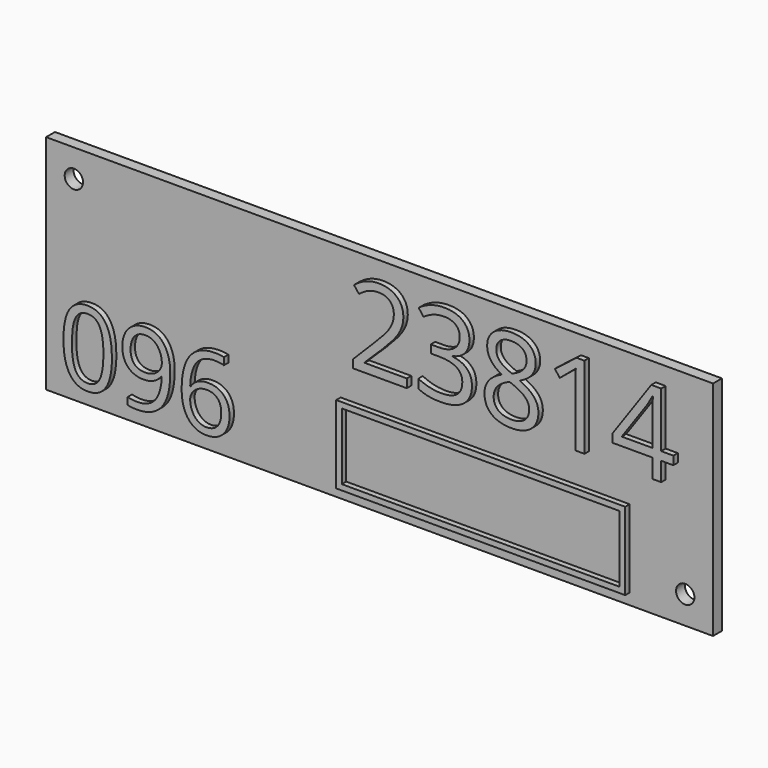
from build123d import *

# Parameters (mm, degrees)
F0_W         = 120
F0_H         = 40
F1_DEPTH     = 2
F3_D         = 3.3
F4_TEXT_SIZE = 20.6651598321
F5_DEPTH     = 1
F6_TEXT_SIZE = 18.4837545126
F7_DEPTH     = 1
F8_W         = 52
F8_H         = 14
F8_W_2       = 49.99999962
F8_H_2       = 11.99999962
F9_DEPTH     = 1


# Not quite as in the source:
# - Text() gives the source's letters only with a copy of the font that has no kerning and outlines rounded to 1/6400 em; it was checked with that copy


with BuildPart() as f1:
    # F0 (on Front) → F1 (new body)
    with BuildSketch(Plane.XZ):
        Rectangle(F0_W, F0_H)
    extrude(amount=F1_DEPTH)

    # F3 (through all)
    with Locations(Plane.XZ.offset(2)):
        with Locations((-55, 15), (55, -15)):
            Hole(F3_D / 2)

    # F4 (on face) → F5 (join)
    with BuildSketch(Plane.XZ.offset(2)):
        with Locations((-5, 2)):
            Text('23814', F4_TEXT_SIZE, font='Open Sans', text_align=(TextAlign.LEFT, TextAlign.BOTTOM))
    extrude(amount=F5_DEPTH)

    # F6 (on face) → F7 (join)
    with BuildSketch(Plane.XZ.offset(2)):
        with Locations((-57, -17)):
            Text('096', F6_TEXT_SIZE, font='Open Sans', text_align=(TextAlign.LEFT, TextAlign.BOTTOM))
    extrude(amount=F7_DEPTH)

    # F8 (on face) → F9 (join)
    with BuildSketch(Plane.XZ.offset(2)):
        with Locations((19, -11)):
            Rectangle(F8_W, F8_H)
        with Locations((19, -11)):
            Rectangle(F8_W_2, F8_H_2, mode=Mode.SUBTRACT)
    extrude(amount=F9_DEPTH)


solid = f1.part
